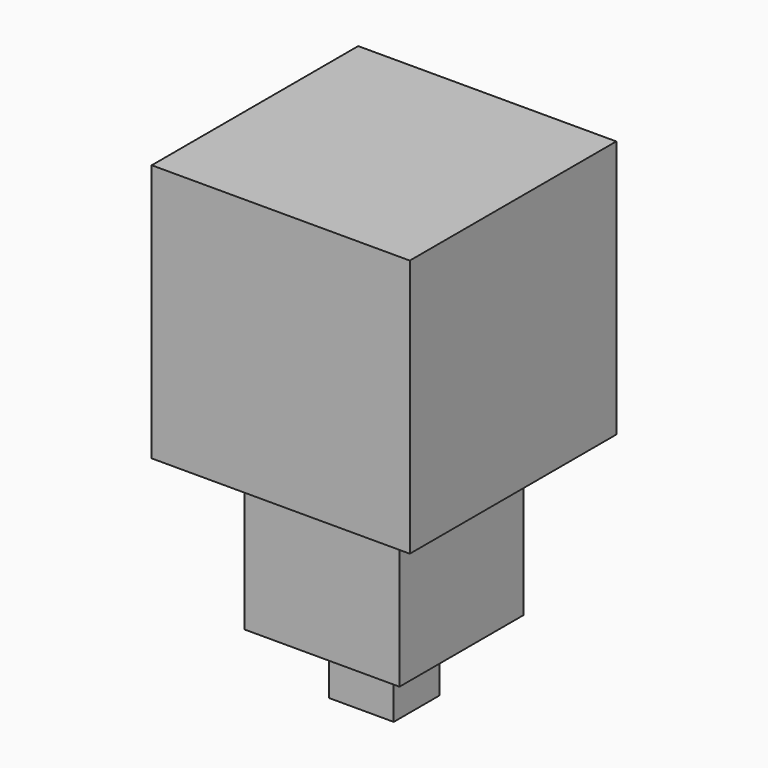
from build123d import *

# Parameters (mm, degrees)
F0_W      = 100
F0_H      = 100
F1_DEPTH  = 100
F2_W      = 21.2592259049
F2_H      = 13.5286012664
F3_DEPTH  = 20
F4_W      = 60
F4_H      = 60
F5_DEPTH  = 60
F7_W      = 35
F7_H      = 27.0690375748
F6_W      = 60
F6_H      = 60
F9_DEPTH  = 100
F10_W     = 25.1245461404
F10_H     = 22.2255568951
F12_DEPTH = 25


# Not quite as in the source:
# - a feature of the source that left no trace in its solid (it failed there, or was rolled back) is left out


with BuildPart() as f1:
    # F0 (on Top) → F1 (new body)
    with BuildSketch(Plane.XY):
        Rectangle(F0_W, F0_H)
    extrude(amount=F1_DEPTH)

    # F2 (on Top) → F3 (join)
    with BuildSketch(Plane.XY):
        Rectangle(F2_W, F2_H)
    extrude(amount=-F3_DEPTH)

    # F4 (on Top) → F5 (join)
    with BuildSketch(Plane.XY):
        Rectangle(F4_W, F4_H)
    extrude(amount=-F5_DEPTH)

    # F7 (on face) + F6 (on face) → F9 (join)
    with BuildSketch(Plane(origin=(0, 0, -60), x_dir=(1, 0, 0), z_dir=(0, 0, -1))):
        Rectangle(F7_W, F7_H)
    with BuildSketch(Plane(origin=(0, 0, -60), x_dir=(1, 0, 0), z_dir=(0, 0, -1))):
        Rectangle(F6_W, F6_H)
    extrude(amount=-F9_DEPTH)

    # F10 (on face) → F12 (join)
    with BuildSketch(Plane(origin=(0, 0, -60), x_dir=(1, 0, 0), z_dir=(0, 0, -1))):
        with Locations((0.4831599072, 0.4831608385)):
            Rectangle(F10_W, F10_H)
    extrude(amount=F12_DEPTH)


solid = f1.part
